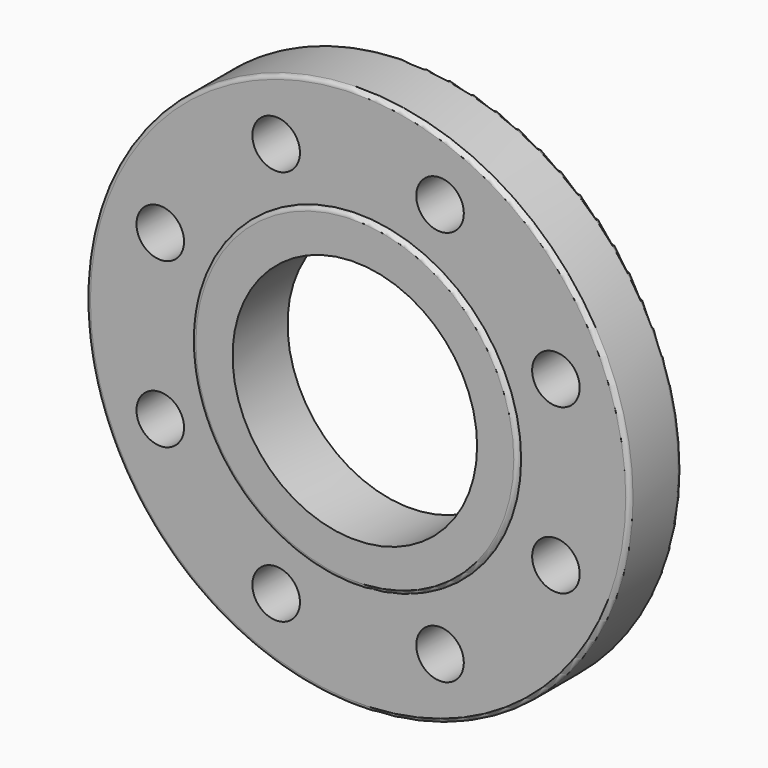
from build123d import *

# Parameters (mm, degrees)
F0_R     = 127
F0_R_2   = 11.1125
F0_R_3   = 57.15
F1_DEPTH = 30.226
F2_R     = 76.2
F2_R_2   = 57.15
F3_DEPTH = 1.905
F4_R     = 1.90499


# Not quite as in the source:
# - a fillet or chamfer is up to 0.001 mm smaller than in the source, because OpenCascade refuses the exact size


with BuildPart() as f1:
    # F0 (on Front) → F1 (new body)
    with BuildSketch(Plane.XZ):
        Circle(F0_R)
        with Locations((-38.2974271774, -92.4581680956)):
            Circle(F0_R_2, mode=Mode.SUBTRACT)
        with Locations((-92.4581680956, -38.2974271774)):
            Circle(F0_R_2, mode=Mode.SUBTRACT)
        with Locations((38.2974271774, -92.4581680956)):
            Circle(F0_R_2, mode=Mode.SUBTRACT)
        with Locations((92.4581680956, -38.2974271774)):
            Circle(F0_R_2, mode=Mode.SUBTRACT)
        with Locations((-92.4581680956, 38.2974271774)):
            Circle(F0_R_2, mode=Mode.SUBTRACT)
        with Locations((-38.2974271774, 92.4581680956)):
            Circle(F0_R_2, mode=Mode.SUBTRACT)
        Circle(F0_R_3, mode=Mode.SUBTRACT)
        with Locations((92.4581680956, 38.2974271774)):
            Circle(F0_R_2, mode=Mode.SUBTRACT)
        with Locations((38.2974271774, 92.4581680956)):
            Circle(F0_R_2, mode=Mode.SUBTRACT)
    extrude(amount=F1_DEPTH)

    # F2 (on face) → F3 (join)
    with BuildSketch(Plane.XZ.offset(30.226)):
        Circle(F2_R)
        Circle(F2_R_2, mode=Mode.SUBTRACT)
    extrude(amount=F3_DEPTH)

    # F4 (radius 1.905 in the source; OpenCascade refuses exactly that, so slightly less here)
    f4_edges = [f1.edges().sort_by_distance(p)[0] for p in [
        (-127, 0, 0),
        (-127, -30.226, 0),
        (-76.2, -32.131, 0),
    ]]
    fillet(f4_edges, radius=F4_R)


solid = f1.part
